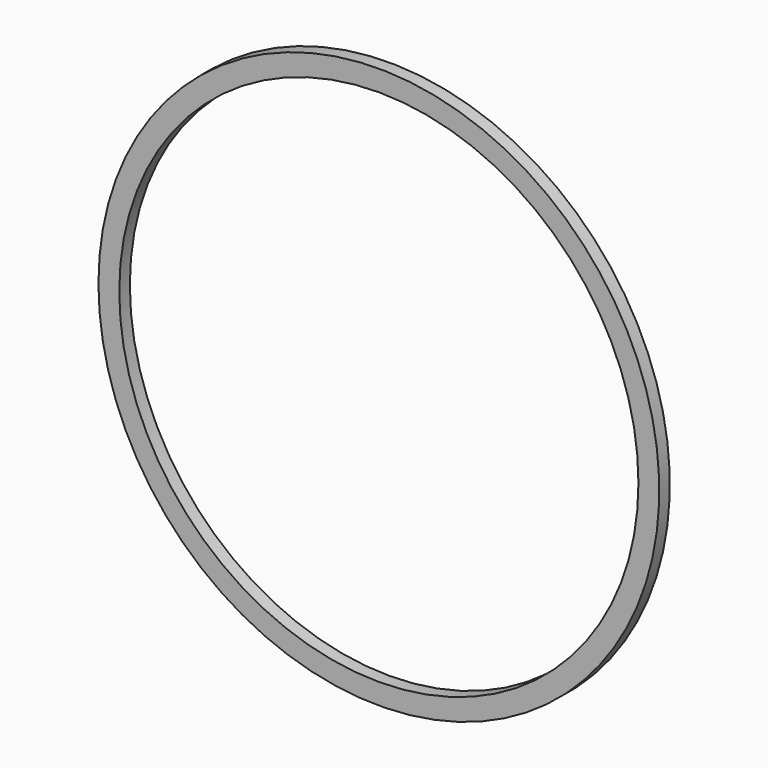
from build123d import *

# Parameters (mm, degrees)
F0_W = 1.486
F0_H = 0.943


# Not quite as in the source:
# - the program builds the solid bodies; features that only make, move or delete a surface that nothing else refers to are left out


with BuildPart() as f2:
    # F0 (on Top) → F2 (revolve)
    with BuildSketch(Plane.XY):
        with Locations((-19.257, 21.2382662386)):
            Rectangle(F0_W, F0_H)
    revolve(axis=Axis((0, 37.5, 0), (0, 1, 0)))


solid = f2.part
